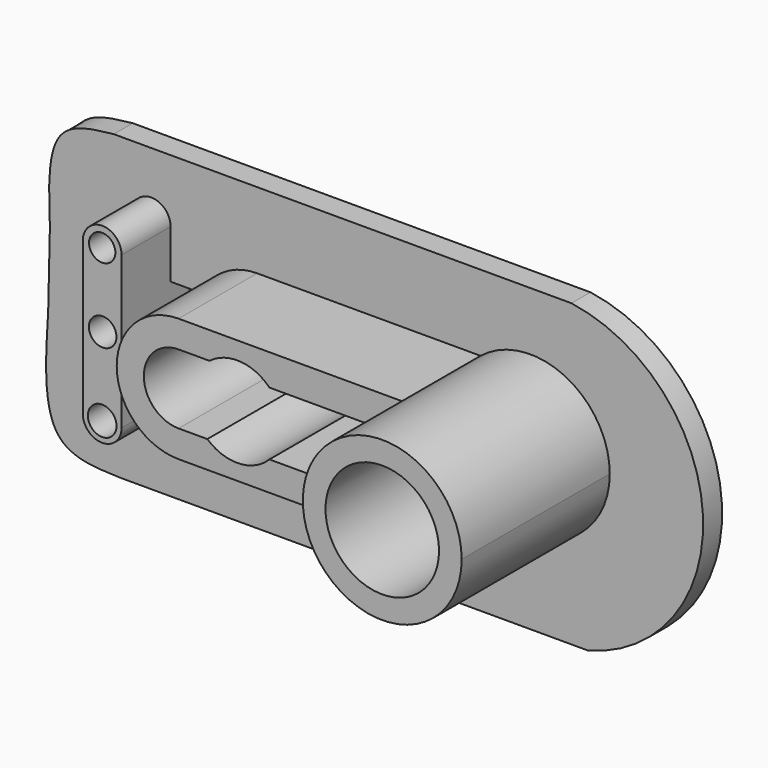
from build123d import *

# Parameters (mm, degrees)
F0_R     = 4.2795303883
F0_R_2   = 4.1203882692
F0_R_3   = 3.9334600098
F1_DEPTH = 25.4
F0_R_4   = 16.9610161395
F2_DEPTH = 62.39313
F3_DEPTH = 36.43448
F6_DEPTH = 7.09099


# Not quite as in the source:
# - the program builds the solid bodies; features that only make, move or delete a surface that nothing else refers to are left out


with BuildPart() as f1:
    # F0 (on Front) → F1 (new body)
    with BuildSketch(Plane.XZ):
        with BuildLine():
            ThreePointArc((-53.0043460473, 28.996894532), (-58.7955482348, 34.7880967196), (-64.5867504224, 28.996894532))
            Line((-64.5867504224, 28.996894532), (-64.5867504224, -16.7940031503))
            ThreePointArc((-64.5867504224, -16.7940031503), (-58.6639644209, -22.3174121933), (-53.0043460473, -16.5246441726))
            Line((-53.0043460473, -16.5246441726), (-53.0043460473, -1.2275470406))
            Line((-53.0043460473, -1.2275470406), (-53.0043460473, 14.5105786386))
            Line((-53.0043460473, 14.5105786386), (-53.0043460473, 28.996894532))
        make_face()
        with Locations((-58.7986803245, -16.5246441726)):
            Circle(F0_R, mode=Mode.SUBTRACT)
        with Locations((-58.6573071778, 6.9124489091)):
            Circle(F0_R_2, mode=Mode.SUBTRACT)
        with Locations((-58.7955482348, 28.996894532)):
            Circle(F0_R_3, mode=Mode.SUBTRACT)
    extrude(amount=F1_DEPTH)


with BuildPart() as f2:
    # F0 (on Front) → F2 (new body)
    with BuildSketch(Plane.XZ):
        with BuildLine():
            ThreePointArc((78.2053648656, 6.6415158399), (64.7229791348, 28.0435082172), (39.5973620512, 25.1240272913))
            ThreePointArc((39.5973620512, 25.1240272913), (35.5176279372, 20.9084727793), (32.5968303911, 15.8208336432))
            ThreePointArc((32.5968303911, 15.8208336432), (30.7511872282, 6.348009445), (32.8305982139, -3.0762595944))
            ThreePointArc((32.8305982139, -3.0762595944), (35.6955553778, -7.8588744416), (39.5973620512, -11.8409956114))
            ThreePointArc((39.5973620512, -11.8409956114), (64.7229791348, -14.7604765374), (78.2053648656, 6.6415158399))
        make_face()
        with Locations((54.4773683713, 6.6415158399)):
            Circle(F0_R_4, mode=Mode.SUBTRACT)
    extrude(amount=F2_DEPTH)

    # F0 (on Front) → F3 (join)
    with BuildSketch(Plane.XZ):
        with BuildLine():
            ThreePointArc((-27.1416550456, 25.1240272913), (-37.0452702112, 22.246695635), (-43.8653233361, 14.5105786386))
            ThreePointArc((-43.8653233361, 14.5105786386), (-45.6241665379, 6.641515799), (-43.8653233361, -1.2275470406))
            ThreePointArc((-43.8653233361, -1.2275470406), (-37.0460046869, -8.9631978878), (-27.1433948729, -11.8409956114))
            Line((-27.1433948729, -11.8409956114), (39.5973620512, -11.8409956114))
            ThreePointArc((39.5973620512, -11.8409956114), (35.6955553778, -7.8588744416), (32.8305982139, -3.0762595944))
            Line((32.8305982139, -3.0762595944), (0, -3.0762595944))
            ThreePointArc((0, -3.0762595944), (-9.1401495961, -7.1109009087), (-18.5496408035, -3.752011153))
            Line((-18.5496408035, -3.752011153), (-27.1371953138, -3.752011153))
            ThreePointArc((-27.1371953138, -3.752011153), (-37.5307223067, 6.6415158399), (-27.1371953138, 17.0350428328))
            Line((-27.1371953138, 17.0350428328), (-17.8983315824, 17.0350428328))
            ThreePointArc((-17.8983315824, 17.0350428328), (-8.7181364976, 19.8334790106), (0, 15.8208336432))
            Line((0, 15.8208336432), (32.5968303911, 15.8208336432))
            ThreePointArc((32.5968303911, 15.8208336432), (35.5176279372, 20.9084727793), (39.5973620512, 25.1240272913))
            Line((39.5973620512, 25.1240272913), (-27.1416550456, 25.1240272913))
        make_face()
    extrude(amount=F3_DEPTH)


with BuildPart() as f6:
    # F0 (on Front) → F6 (new body)
    with BuildSketch(Plane.XZ):
        with BuildLine():
            Line((-68.2164430618, -41.9541485608), (71.6157257557, -41.9541485608))
            ThreePointArc((71.6157257557, -41.9541485608), (106.0450219063, 4.9024018867), (66.7851641774, 47.7926842868))
            Line((66.7851641774, 47.7926842868), (-69.9961259961, 47.7926842868))
            add(Edge.make_bspline(
                [(-69.9961259961, 47.7926842868), (-76.2263024319, 47.1345590327), (-90.1510844896, 45.6636134143), (-89.4510040109, 27.3845536081), (-89.0641510487, 17.2838456929)],
                knots=[0, 0, 0, 0, 0.4474164414, 1, 1, 1, 1], degree=3))
            Line((-89.0641510487, 17.2838456929), (-89.5726308227, -4.835061729))
            add(Edge.make_bspline(
                [(-68.2164430618, -41.9541485608), (-75.3510688203, -41.7581987898), (-91.8886893642, -41.3039993589), (-90.4121593424, -18.0543792359), (-89.5726308227, -4.835061729)],
                knots=[0, 0, 0, 0, 0.4314179141, 1, 1, 1, 1], degree=3))
        make_face()
        with BuildLine():
            Line((-64.5867504224, -16.7940031503), (-64.5867504224, 28.996894532))
            ThreePointArc((-64.5867504224, 28.996894532), (-58.7955482348, 34.7880967196), (-53.0043460473, 28.996894532))
            Line((-53.0043460473, 28.996894532), (-53.0043460473, 14.5105786386))
            Line((-53.0043460473, 14.5105786386), (-43.8653233361, 14.5105786386))
            ThreePointArc((-43.8653233361, 14.5105786386), (-37.0452702112, 22.246695635), (-27.1416550456, 25.1240272913))
            Line((-27.1416550456, 25.1240272913), (39.5973620512, 25.1240272913))
            ThreePointArc((39.5973620512, 25.1240272913), (64.7229791348, 28.0435082172), (78.2053648656, 6.6415158399))
            ThreePointArc((78.2053648656, 6.6415158399), (64.7229791348, -14.7604765374), (39.5973620512, -11.8409956114))
            Line((39.5973620512, -11.8409956114), (-27.1433948729, -11.8409956114))
            ThreePointArc((-27.1433948729, -11.8409956114), (-37.0460046869, -8.9631978878), (-43.8653233361, -1.2275470406))
            Line((-43.8653233361, -1.2275470406), (-53.0043460473, -1.2275470406))
            Line((-53.0043460473, -1.2275470406), (-53.0043460473, -16.5246441726))
            ThreePointArc((-53.0043460473, -16.5246441726), (-58.6639644209, -22.3174121933), (-64.5867504224, -16.7940031503))
        make_face(mode=Mode.SUBTRACT)
    extrude(amount=F6_DEPTH)


solid = Compound([f1.part, f2.part, f6.part])
